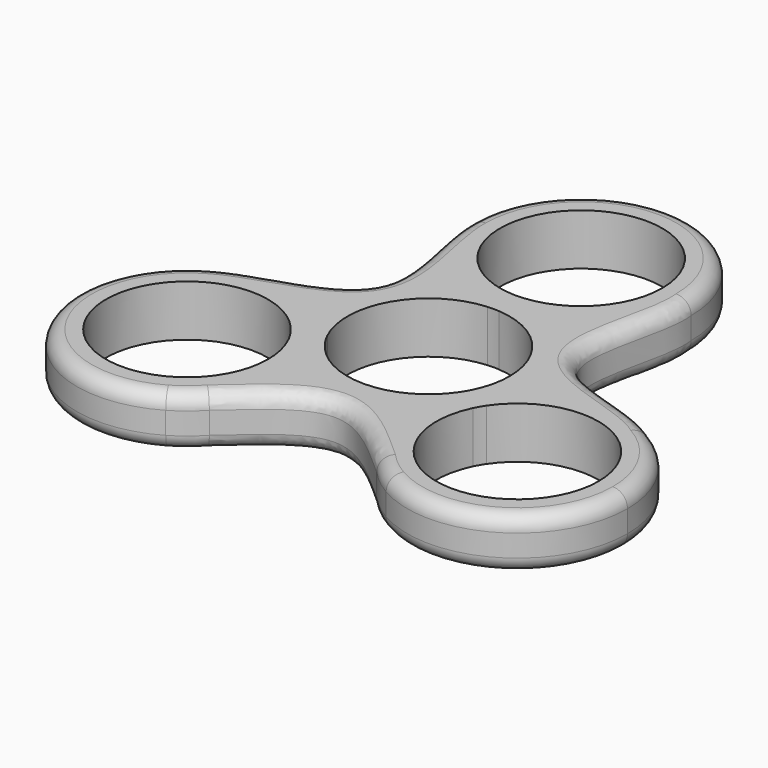
from build123d import *

# Parameters (mm, degrees)
F1_DEPTH = 7
F2_R     = 2
F3_R     = 1.9999


# Not quite as in the source:
# - a fillet or chamfer is up to 0.001 mm smaller than in the source, because OpenCascade refuses the exact size


with BuildPart() as f1:
    # F0 (on Top) → F1 (new body)
    with BuildSketch(Plane.XY):
        with BuildLine():
            ThreePointArc((15, 26), (12.9855635535, 18.4916620216), (7.4833147735, 13))
            ThreePointArc((7.4833147735, 13), (12.9855635535, 7.5083379784), (15, 0))
            ThreePointArc((15, 0), (14.999996909, -0.0096296528), (14.999987636, -0.0192593016))
            ThreePointArc((14.999987636, -0.0192593016), (22.5070308456, 1.999996909), (30.0166604984, -0.0096189432))
            add(Edge.make_bspline(
                [(30.0166604984, -0.0096189432), (25.6438055998, 3.2456274247), (7.0745608208, 4.0844995943), (15.6326986009, 20.5853733868), (15, 26)],
                knots=[0, 0, 0, 0, 0.5, 1, 1, 1, 1], degree=3))
        make_face()
        with BuildLine():
            ThreePointArc((0.7972503815, 14.9787980769), (4.2568592036, 14.3832941193), (7.4833147735, 13))
            ThreePointArc((7.4833147735, 13), (12.9855635535, 18.4916620216), (15, 26))
            ThreePointArc((15, 26), (0, 41), (-15, 26))
            ThreePointArc((-15, 26), (-12.9855635535, 18.4916620216), (-7.4833147735, 13))
            ThreePointArc((-7.4833147735, 13), (-4.2568592036, 14.3832941193), (-0.7972503815, 14.9787980769))
            ThreePointArc((-0.7972503815, 14.9787980769), (-7.5263830385, 34.0904918489), (11.05, 26))
            ThreePointArc((11.05, 26), (8.0904918489, 18.4736169615), (0.7972503815, 14.9787980769))
        make_face()
        with BuildLine():
            ThreePointArc((30.0166604984, -0.0096189432), (22.5070308456, 1.999996909), (14.999987636, -0.0192593016))
            ThreePointArc((14.999987636, -0.0192593016), (14.5847276992, -3.505098849), (13.3706448435, -6.7989599549))
            ThreePointArc((13.3706448435, -6.7989599549), (25.7600404494, -2.4367151656), (33.5666604984, -13))
            ThreePointArc((33.5666604984, -13), (20.0438675129, -23.7697629895), (12.573394462, -8.179838122))
            ThreePointArc((12.573394462, -8.179838122), (10.3278684956, -10.8781952702), (7.5166728624, -12.9807406984))
            ThreePointArc((7.5166728624, -12.9807406984), (8.5199026945, -18.3935860964), (11.4083630139, -23.0799666168))
            add(Edge.make_bspline(
                [(11.4083630139, -23.0799666168), (12.6111288421, -24.134869858), (13.8138946702, -25.1488195737), (15.0166604984, -25.9903810568)],
                knots=[0.8798568602, 0.8798568602, 0.8798568602, 0.8798568602, 1, 1, 1, 1], degree=3))
            ThreePointArc((15.0166604984, -25.9903810568), (30.0166604984, -25.9903810568), (37.5166604984, -13))
            ThreePointArc((37.5166604984, -13), (35.5070415552, -5.5), (30.0166604984, -0.0096189432))
        make_face()
        with BuildLine():
            ThreePointArc((-14.999987636, -0.0192593016), (-12.9903810568, 7.5), (-7.4833147735, 13))
            ThreePointArc((-7.4833147735, 13), (-12.9855635535, 18.4916620216), (-15, 26))
            add(Edge.make_bspline(
                [(-30.0166604984, -0.0096189432), (-25.2041229475, 2.991776527), (-7.5142434731, 4.3383504919), (-15.1930159486, 20.3315224891), (-15, 26)],
                knots=[0, 0, 0, 0, 0.5, 1, 1, 1, 1], degree=3))
            ThreePointArc((-30.0166604984, -0.0096189432), (-22.5070308456, 1.999996909), (-14.999987636, -0.0192593016))
        make_face()
        with BuildLine():
            ThreePointArc((11.4083630139, -23.0799666168), (8.5199026945, -18.3935860964), (7.5166728624, -12.9807406984))
            ThreePointArc((7.5166728624, -12.9807406984), (0, -15), (-7.5166728624, -12.9807406984))
            ThreePointArc((-7.5166728624, -12.9807406984), (-7.5166635894, -12.9903703472), (-7.5166604984, -13))
            ThreePointArc((-7.5166604984, -13), (-8.5233681362, -18.4025705795), (-11.4083630139, -23.0799666168))
            add(Edge.make_bspline(
                [(-11.4083630139, -23.0799666168), (-7.6055753426, -19.7446764498), (0, -12.2553235502), (7.6055753426, -19.7446764498), (11.4083630139, -23.0799666168)],
                knots=[0.1201431398, 0.1201431398, 0.1201431398, 0.1201431398, 0.5, 0.8798568602, 0.8798568602, 0.8798568602, 0.8798568602], degree=3))
        make_face()
        with BuildLine():
            ThreePointArc((-13.3706448435, -6.7989599549), (-14.5847276992, -3.505098849), (-14.999987636, -0.0192593016))
            ThreePointArc((-14.999987636, -0.0192593016), (-22.5070308456, 1.999996909), (-30.0166604984, -0.0096189432))
            ThreePointArc((-30.0166604984, -0.0096189432), (-35.5070415552, -20.5), (-15.0166604984, -25.9903810568))
            add(Edge.make_bspline(
                [(-15.0166604984, -25.9903810568), (-13.8138946702, -25.1488195737), (-12.6111288421, -24.134869858), (-11.4083630139, -23.0799666168)],
                knots=[0, 0, 0, 0, 0.1201431398, 0.1201431398, 0.1201431398, 0.1201431398], degree=3))
            ThreePointArc((-11.4083630139, -23.0799666168), (-8.5233681362, -18.4025705795), (-7.5166604984, -13))
            ThreePointArc((-7.5166604984, -13), (-7.5166635894, -12.9903703472), (-7.5166728624, -12.9807406984))
            ThreePointArc((-7.5166728624, -12.9807406984), (-10.3278684956, -10.8781952702), (-12.573394462, -8.179838122))
            ThreePointArc((-12.573394462, -8.179838122), (-11.7468975089, -10.5272070145), (-11.4666604984, -13))
            ThreePointArc((-11.4666604984, -13), (-33.0799453328, -16.243379951), (-13.3706448435, -6.7989599549))
        make_face()
        with BuildLine():
            add(Edge.make_bspline(
                [(11.4083630139, -23.0799666168), (12.6111288421, -24.134869858), (13.8138946702, -25.1488195737), (15.0166604984, -25.9903810568)],
                knots=[0.8798568602, 0.8798568602, 0.8798568602, 0.8798568602, 1, 1, 1, 1], degree=3))
            ThreePointArc((11.4083630139, -23.0799666168), (13.0993991199, -24.6754095487), (15.0166604984, -25.9903810568))
        make_face()
        with BuildLine():
            ThreePointArc((-15.0166604984, -25.9903810568), (-13.0993991199, -24.6754095487), (-11.4083630139, -23.0799666168))
            add(Edge.make_bspline(
                [(-15.0166604984, -25.9903810568), (-13.8138946702, -25.1488195737), (-12.6111288421, -24.134869858), (-11.4083630139, -23.0799666168)],
                knots=[0, 0, 0, 0, 0.1201431398, 0.1201431398, 0.1201431398, 0.1201431398], degree=3))
        make_face()
        with BuildLine():
            ThreePointArc((-9.1460156549, -6.2010400451), (-9.5695807118, -5.525), (-9.9432660364, -4.820161878))
            ThreePointArc((-9.9432660364, -4.820161878), (-12.1887920028, -2.1218047298), (-14.999987636, -0.0192593016))
            ThreePointArc((-14.999987636, -0.0192593016), (-14.5847276992, -3.505098849), (-13.3706448435, -6.7989599549))
            ThreePointArc((-13.3706448435, -6.7989599549), (-12.9470797866, -7.475), (-12.573394462, -8.179838122))
            ThreePointArc((-12.573394462, -8.179838122), (-10.3278684956, -10.8781952702), (-7.5166728624, -12.9807406984))
            ThreePointArc((-7.5166728624, -12.9807406984), (-7.9319327992, -9.494901151), (-9.1460156549, -6.2010400451))
        make_face()
        with BuildLine():
            ThreePointArc((7.5166728624, -12.9807406984), (7.9319327992, -9.494901151), (9.1460156549, -6.2010400451))
            ThreePointArc((9.1460156549, -6.2010400451), (0, -11.05), (-9.1460156549, -6.2010400451))
            ThreePointArc((-9.1460156549, -6.2010400451), (-7.9319327992, -9.494901151), (-7.5166728624, -12.9807406984))
            ThreePointArc((-7.5166728624, -12.9807406984), (0, -15), (7.5166728624, -12.9807406984))
        make_face()
        with BuildLine():
            ThreePointArc((14.999987636, -0.0192593016), (12.1887920028, -2.1218047298), (9.9432660364, -4.820161878))
            ThreePointArc((9.9432660364, -4.820161878), (9.5695807118, -5.525), (9.1460156549, -6.2010400451))
            ThreePointArc((9.1460156549, -6.2010400451), (7.9319327992, -9.494901151), (7.5166728624, -12.9807406984))
            ThreePointArc((7.5166728624, -12.9807406984), (10.3278684956, -10.8781952702), (12.573394462, -8.179838122))
            ThreePointArc((12.573394462, -8.179838122), (12.9470797866, -7.475), (13.3706448435, -6.7989599549))
            ThreePointArc((13.3706448435, -6.7989599549), (14.5847276992, -3.505098849), (14.999987636, -0.0192593016))
        make_face()
        with BuildLine():
            ThreePointArc((0.7972503815, 11.0212019231), (8.0904918489, 7.5263830385), (11.05, 0))
            ThreePointArc((11.05, 0), (10.7697629895, -2.4727929855), (9.9432660364, -4.820161878))
            ThreePointArc((9.9432660364, -4.820161878), (12.1887920028, -2.1218047298), (14.999987636, -0.0192593016))
            ThreePointArc((14.999987636, -0.0192593016), (14.999996909, -0.0096296528), (15, 0))
            ThreePointArc((15, 0), (12.9855635535, 7.5083379784), (7.4833147735, 13))
            ThreePointArc((7.4833147735, 13), (4.2568592036, 11.6167058807), (0.7972503815, 11.0212019231))
        make_face()
        with BuildLine():
            ThreePointArc((-0.7972503815, 11.0212019231), (0, 11.05), (0.7972503815, 11.0212019231))
            ThreePointArc((0.7972503815, 11.0212019231), (4.2568592036, 11.6167058807), (7.4833147735, 13))
            ThreePointArc((7.4833147735, 13), (4.2568592036, 14.3832941193), (0.7972503815, 14.9787980769))
            ThreePointArc((0.7972503815, 14.9787980769), (0, 14.95), (-0.7972503815, 14.9787980769))
            ThreePointArc((-0.7972503815, 14.9787980769), (-4.2568592036, 14.3832941193), (-7.4833147735, 13))
            ThreePointArc((-7.4833147735, 13), (-4.2568592036, 11.6167058807), (-0.7972503815, 11.0212019231))
        make_face()
        with BuildLine():
            ThreePointArc((-9.9432660364, -4.820161878), (-9.5695807118, 5.525), (-0.7972503815, 11.0212019231))
            ThreePointArc((-0.7972503815, 11.0212019231), (-4.2568592036, 11.6167058807), (-7.4833147735, 13))
            ThreePointArc((-7.4833147735, 13), (-12.9903810568, 7.5), (-14.999987636, -0.0192593016))
            ThreePointArc((-14.999987636, -0.0192593016), (-12.1887920028, -2.1218047298), (-9.9432660364, -4.820161878))
        make_face()
    extrude(amount=F1_DEPTH)

    # F2
    f2_edges = [f1.edges().sort_by_distance(p)[0] for p in [
        (-13.856406, 8, 7),
        (0, -16, 7),
        (13.856406, 8, 7),
        (0, 41, 7),
        (34.19207, -22.417261, 7),
        (-34.19207, -22.417261, 7),
    ]]
    fillet(f2_edges, radius=F2_R)

    # F3 (radius 2 in the source; OpenCascade refuses exactly that, so slightly less here)
    f3_edges = [f1.edges().sort_by_distance(p)[0] for p in [
        (0, -16, 0),
        (-13.856406, 8, 0),
        (13.856406, 8, 0),
        (34.19207, -22.417261, 0),
        (0, 41, 0),
        (-34.19207, -22.417261, 0),
    ]]
    fillet(f3_edges, radius=F3_R)


solid = f1.part
